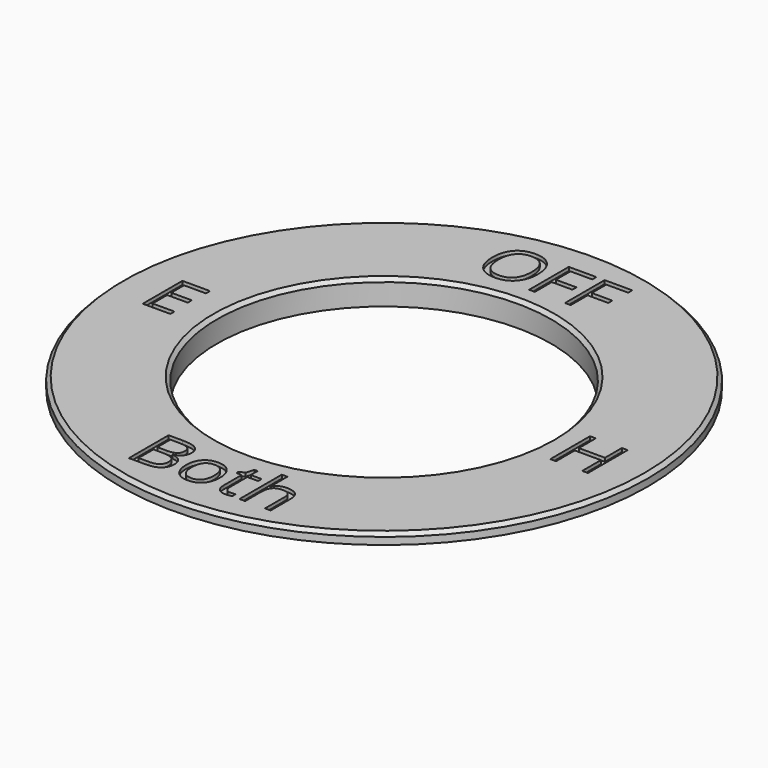
from build123d import *

# Parameters (mm, degrees)
F0_R         = 73.8815367264
F0_R_2       = 46.75
F1_DEPTH     = 3
F2_R         = 48
F2_R_2       = 46.75
F3_DEPTH     = 4
F4_TEXT_SIZE = 19.4444444444
F5_DEPTH     = 1
F6_SIZE      = 1


# Not quite as in the source:
# - Text() gives the source's letters only with a copy of the font that has no kerning and outlines rounded to 1/6400 em; it was checked with that copy


with BuildPart() as f1:
    # F0 (on Top) → F1 (new body)
    with BuildSketch(Plane.XY):
        Circle(F0_R)
        Circle(F0_R_2, mode=Mode.SUBTRACT)
    extrude(amount=F1_DEPTH)

    # F2 (on face) → F3 (join)
    with BuildSketch(Plane(origin=(0, 0, 0), x_dir=(1, 0, 0), z_dir=(0, 0, -1))):
        Circle(F2_R)
        Circle(F2_R_2, mode=Mode.SUBTRACT)
    extrude(amount=F3_DEPTH)

    # F4 (on face) → F5 (cut)
    with BuildSketch(Plane.XY.offset(3)):
        with Locations((-18.0423177083, 51.9770115369)):
            Text('OFF', F4_TEXT_SIZE, font='Open Sans', text_align=(TextAlign.LEFT, TextAlign.BOTTOM))
        with Locations((-21.4192708333, -64.9000856041)):
            Text('Both', F4_TEXT_SIZE, font='Open Sans', text_align=(TextAlign.LEFT, TextAlign.BOTTOM))
        with Locations((-64.7179113398, -5.9423797647)):
            Text('E', F4_TEXT_SIZE, font='Open Sans', text_align=(TextAlign.LEFT, TextAlign.BOTTOM))
        with Locations((50.7977884263, -7.7231072427)):
            Text('H', F4_TEXT_SIZE, font='Open Sans', text_align=(TextAlign.LEFT, TextAlign.BOTTOM))
    extrude(amount=-F5_DEPTH, mode=Mode.SUBTRACT)

    # F6
    f6_edges = [f1.edges().sort_by_distance(p)[0] for p in [
        (-73.881537, 0, 3),
        (-46.75, 0, 3),
        (-48, 0, -4),
    ]]
    chamfer(f6_edges, length=F6_SIZE)


solid = f1.part
